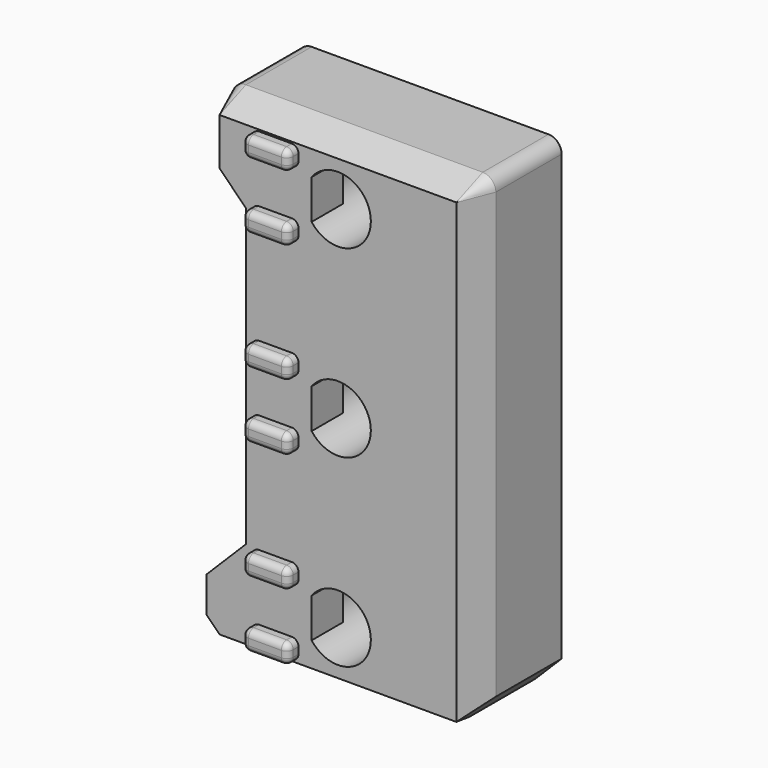
from build123d import *

# Parameters (mm, degrees)
F1_DEPTH    = 6
F2_DEPTH    = 11.5
F3_SIZE     = 4
F4_W        = 6
F4_H        = 45
F5_DEPTH    = 25
F6_SIZE     = 5.99999
F8_START    = -6
F7_W        = 2
F7_H        = 3
F8_DEPTH    = 7
F9_R        = 1
F10_R       = 1
F11_R       = 2
F12_SIZE2   = 2
F12_SIZE    = 5
F12_2_SIZE2 = 2
F12_2_SIZE  = 5
F13_W       = 3
F13_H       = 7
F14_DEPTH   = 4


# Not quite as in the source:
# - a fillet or chamfer is up to 0.001 mm smaller than in the source, because OpenCascade refuses the exact size


with BuildPart() as f1:
    # F0 (on Front) → F1 (new body)
    with BuildSketch(Plane.XZ):
        with BuildLine():
            Line((-4, 36.76), (-20, 36.76))
            Line((-20, 36.76), (-20, -36.76))
            Line((-20, -36.76), (-4, -36.76))
            Line((-4, -36.76), (-4, -31))
            ThreePointArc((-4, -31), (-5, -28), (-4, -25))
            Line((-4, -25), (-4, -3))
            ThreePointArc((-4, -3), (-5, 0), (-4, 3))
            Line((-4, 3), (-4, 25))
            ThreePointArc((-4, 25), (-5, 28), (-4, 31))
            Line((-4, 31), (-4, 36.76))
        make_face()
        with BuildLine():
            Line((20, 36.76), (-4, 36.76))
            Line((-4, 36.76), (-4, 31))
            ThreePointArc((-4, 31), (1.5811388301, 32.7434164903), (5, 28))
            ThreePointArc((5, 28), (1.5811388301, 23.2565835097), (-4, 25))
            Line((-4, 25), (-4, 3))
            ThreePointArc((-4, 3), (1.5811388301, 4.7434164903), (5, 0))
            ThreePointArc((5, 0), (1.5811388301, -4.7434164903), (-4, -3))
            Line((-4, -3), (-4, -25))
            ThreePointArc((-4, -25), (1.5811388301, -23.2565835097), (5, -28))
            ThreePointArc((5, -28), (1.5811388301, -32.7434164903), (-4, -31))
            Line((-4, -31), (-4, -36.76))
            Line((-4, -36.76), (20, -36.76))
            Line((20, -36.76), (20, 36.76))
        make_face()
        with BuildLine():
            Line((-4, 25), (-4, 31))
            ThreePointArc((-4, 31), (-5, 28), (-4, 25))
        make_face()
        with BuildLine():
            Line((-4, -3), (-4, 3))
            ThreePointArc((-4, 3), (-5, 0), (-4, -3))
        make_face()
        with BuildLine():
            ThreePointArc((-4, -25), (-5, -28), (-4, -31))
            Line((-4, -31), (-4, -25))
        make_face()
    extrude(amount=F1_DEPTH)

    # F0 (on Front) → F2 (join)
    with BuildSketch(Plane.XZ):
        with BuildLine():
            Line((20, 36.76), (-4, 36.76))
            Line((-4, 36.76), (-4, 31))
            ThreePointArc((-4, 31), (1.5811388301, 32.7434164903), (5, 28))
            ThreePointArc((5, 28), (1.5811388301, 23.2565835097), (-4, 25))
            Line((-4, 25), (-4, 3))
            ThreePointArc((-4, 3), (1.5811388301, 4.7434164903), (5, 0))
            ThreePointArc((5, 0), (1.5811388301, -4.7434164903), (-4, -3))
            Line((-4, -3), (-4, -25))
            ThreePointArc((-4, -25), (1.5811388301, -23.2565835097), (5, -28))
            ThreePointArc((5, -28), (1.5811388301, -32.7434164903), (-4, -31))
            Line((-4, -31), (-4, -36.76))
            Line((-4, -36.76), (20, -36.76))
            Line((20, -36.76), (20, 36.76))
        make_face()
        with BuildLine():
            Line((-4, 36.76), (-20, 36.76))
            Line((-20, 36.76), (-20, -36.76))
            Line((-20, -36.76), (-4, -36.76))
            Line((-4, -36.76), (-4, -31))
            ThreePointArc((-4, -31), (-5, -28), (-4, -25))
            Line((-4, -25), (-4, -3))
            ThreePointArc((-4, -3), (-5, 0), (-4, 3))
            Line((-4, 3), (-4, 25))
            ThreePointArc((-4, 25), (-5, 28), (-4, 31))
            Line((-4, 31), (-4, 36.76))
        make_face()
    extrude(amount=-F2_DEPTH)

    # F3
    f3_edges = [f1.edges().sort_by_distance(p)[0] for p in [
        (20, 2.75, -36.76),
        (-20, 2.75, -36.76),
    ]]
    chamfer(f3_edges, length=F3_SIZE)

    # F4 (on Front) → F5 (cut, symmetric)
    with BuildSketch(Plane.XZ):
        with Locations((-17, 1.1105760932)):
            Rectangle(F4_W, F4_H)
    extrude(amount=F5_DEPTH, both=True, mode=Mode.SUBTRACT)

    # F6 (size 6 in the source; OpenCascade refuses exactly that, so slightly less here)
    f6_edges = [f1.edges().sort_by_distance(p)[0] for p in [
        (-20, 2.75, 23.610576),
        (-20, 2.75, -21.389424),
    ]]
    chamfer(f6_edges, length=F6_SIZE)

    # F7 (on Right) → F8 (join)
    with BuildSketch(Plane.YZ.offset(F8_START)):
        with Locations((-7, 33)):
            Rectangle(F7_W, F7_H)
        with Locations((-7, 23)):
            Rectangle(F7_W, F7_H)
        with Locations((-7, 5)):
            Rectangle(F7_W, F7_H)
        with Locations((-7, -5)):
            Rectangle(F7_W, F7_H)
        with Locations((-7, -23)):
            Rectangle(F7_W, F7_H)
        with Locations((-7, -33)):
            Rectangle(F7_W, F7_H)
    extrude(amount=-F8_DEPTH)

    # F9
    f9_edges = [f1.edges().sort_by_distance(p)[0] for p in [
        (-13, -7, -34.5),
    ]]
    fillet(f9_edges, radius=F9_R)

    # F10
    f10_edges = [f1.edges().sort_by_distance(p)[0] for p in [
        (-6, -7, -34.5),
        (-13, -7, -31.5),
        (-6, -7, -31.5),
        (-9.5, -8, -31.5),
        (-9, -8, -34.5),
        (-6, -8, -33),
        (-6, -7, -24.5),
        (-13, -7, -24.5),
        (-13, -7, -21.5),
        (-6, -7, -21.5),
        (-9.5, -8, -21.5),
        (-9.5, -8, -24.5),
        (-6, -8, -23),
        (-13, -8, -23),
        (-6, -7, -6.5),
        (-13, -7, -6.5),
        (-13, -7, -3.5),
        (-6, -7, -3.5),
        (-9.5, -8, -6.5),
        (-9.5, -8, -3.5),
        (-6, -8, -5),
        (-13, -8, -5),
        (-13, -7, 3.5),
        (-6, -7, 3.5),
        (-6, -7, 6.5),
        (-13, -7, 6.5),
        (-9.5, -8, 6.5),
        (-9.5, -8, 3.5),
        (-13, -8, 5),
        (-6, -8, 5),
        (-13, -7, 21.5),
        (-6, -7, 21.5),
        (-6, -7, 24.5),
        (-13, -7, 24.5),
        (-9.5, -8, 24.5),
        (-9.5, -8, 21.5),
        (-6, -8, 23),
        (-13, -8, 23),
        (-9.5, -8, 31.5),
        (-13, -7, 31.5),
        (-6, -7, 31.5),
        (-6, -8, 33),
        (-13, -8, 33),
        (-9.5, -8, 34.5),
        (-13, -7, 34.5),
        (-6, -7, 34.5),
    ]]
    fillet(f10_edges, radius=F10_R)

    # F11
    f11_edges = [f1.edges().sort_by_distance(p)[0] for p in [
        (-20, 2.75, 36.76),
        (20, 2.75, 36.76),
    ]]
    fillet(f11_edges, radius=F11_R)

    # F12
    f12_edges = [f1.edges().sort_by_distance(p)[0] for p in [
        (20, -6, 1),
    ]]
    f12_side = f1.faces().sort_by_distance((20, 2.75, 1))[0]
    chamfer(f12_edges, length=F12_SIZE, length2=F12_SIZE2, reference=f12_side)

    # F12#2
    f12_2_edges = [f1.edges().sort_by_distance(p)[0] for p in [
        (0, -6, -36.76),
    ]]
    f12_2_side = f1.faces().sort_by_distance((0, 2.75, -36.76))[0]
    chamfer(f12_2_edges, length=F12_2_SIZE, length2=F12_2_SIZE2, reference=f12_2_side)

    # F13 (on face) → F14 (cut)
    with BuildSketch(Plane(origin=(-14, 0, 0), x_dir=(0, -1, 0), z_dir=(-1, 0, 0))):
        with Locations((-8, 12.6105760932)):
            Rectangle(F13_W, F13_H)
        with Locations((-8, -10.3894239068)):
            Rectangle(F13_W, F13_H)
    extrude(amount=-F14_DEPTH, mode=Mode.SUBTRACT)


solid = f1.part
